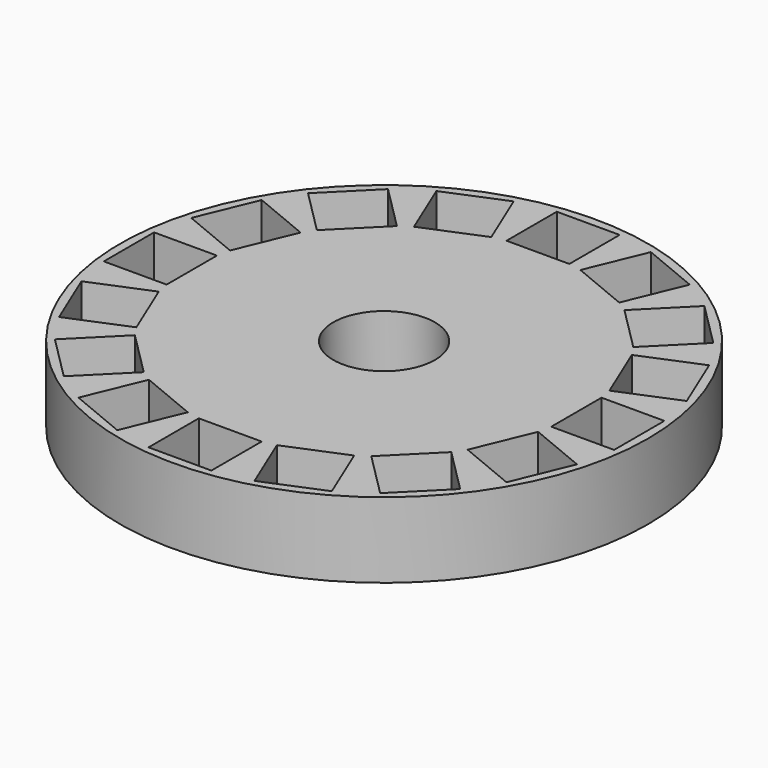
from build123d import *

# Parameters (mm, degrees)
F0_W     = 21
F0_H     = 6
F2_R     = 4.05
F3_DEPTH = 25
F4_W     = 5
F4_H     = 5
F5_DEPTH = 5


# Not quite as in the source:
# - a feature names something its author has since deleted; it is built from what else it names


with BuildPart() as f1:
    # F0 (on Front) → F1 (revolve)
    with BuildSketch(Plane.XZ):
        with Locations((10.5, 3)):
            Rectangle(F0_W, F0_H)
    revolve(axis=Axis((0, 0, 3), (0, 0, -1)))

    # F2 (on Top) → F3 (cut)
    with BuildSketch(Plane.XY):
        Circle(F2_R)
    extrude(amount=F3_DEPTH, mode=Mode.SUBTRACT)

    # F4 (on face) → F5 (cut)
    with BuildSketch(Plane.XY.offset(6)):
        with Locations((0, 17.8)):
            Rectangle(F4_W, F4_H)
        Polygon((3.5453576839, 15.0920654283), (8.1647553465, 13.1786482665), (10.0781725083, 17.7980459291), (5.4587748457, 19.7114630909), align=None)
        Polygon((9.0509667992, 12.5865007051), (12.5865007051, 9.0509667992), (16.1220346111, 12.5865007051), (12.5865007051, 16.1220346111), align=None)
        Polygon((13.1786482665, 8.1647553465), (15.0920654283, 3.5453576839), (19.7114630909, 5.4587748457), (17.7980459291, 10.0781725083), align=None)
        with Locations((17.8, 0)):
            Rectangle(F4_W, F4_H)
        Polygon((15.0920654283, -3.5453576839), (13.1786482665, -8.1647553465), (17.7980459291, -10.0781725083), (19.7114630909, -5.4587748457), align=None)
        Polygon((12.5865007051, -9.0509667992), (9.0509667992, -12.5865007051), (12.5865007051, -16.1220346111), (16.1220346111, -12.5865007051), align=None)
        Polygon((8.1647553465, -13.1786482665), (3.5453576839, -15.0920654283), (5.4587748457, -19.7114630909), (10.0781725083, -17.7980459291), align=None)
        with Locations((0, -17.8)):
            Rectangle(F4_W, F4_H)
        Polygon((-3.5453576839, -15.0920654283), (-8.1647553465, -13.1786482665), (-10.0781725083, -17.7980459291), (-5.4587748457, -19.7114630909), align=None)
        Polygon((-9.0509667992, -12.5865007051), (-12.5865007051, -9.0509667992), (-16.1220346111, -12.5865007051), (-12.5865007051, -16.1220346111), align=None)
        Polygon((-13.1786482665, -8.1647553465), (-15.0920654283, -3.5453576839), (-19.7114630909, -5.4587748457), (-17.7980459291, -10.0781725083), align=None)
        with Locations((-17.8, 0)):
            Rectangle(F4_W, F4_H)
        Polygon((-15.0920654283, 3.5453576839), (-13.1786482665, 8.1647553465), (-17.7980459291, 10.0781725083), (-19.7114630909, 5.4587748457), align=None)
        Polygon((-12.5865007051, 9.0509667992), (-9.0509667992, 12.5865007051), (-12.5865007051, 16.1220346111), (-16.1220346111, 12.5865007051), align=None)
        Polygon((-8.1647553465, 13.1786482665), (-3.5453576839, 15.0920654283), (-5.4587748457, 19.7114630909), (-10.0781725083, 17.7980459291), align=None)
    extrude(amount=-F5_DEPTH, mode=Mode.SUBTRACT)


solid = f1.part
